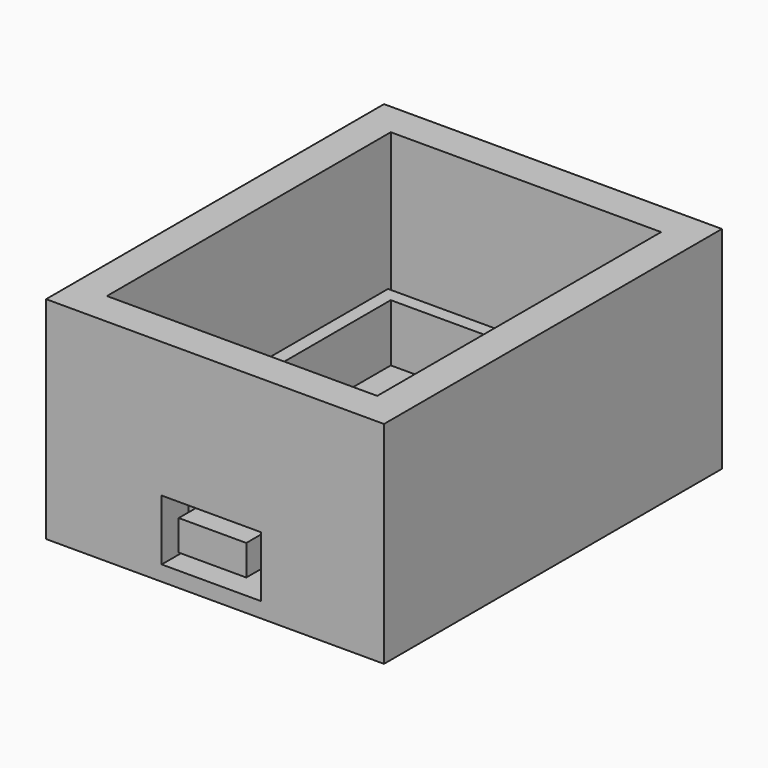
from build123d import *

# Parameters (mm, degrees)
F0_W      = 29.2
F0_H      = 37.7
F1_DEPTH  = 10
F2_T      = -1.6
F3_W      = 8
F3_H      = 3.6
F4_DEPTH  = 1.6
F5_W      = 4
F5_H      = 2.5
F6_DEPTH  = 1.6
F7_W      = 26
F7_H      = 34.5
F8_DEPTH  = 1.6
F9_W      = 32
F9_H      = 4
F9_W_2    = 4
F9_H_2    = 42
F10_DEPTH = 25
F11_W     = 40
F11_H     = 50
F11_W_2   = 32
F11_H_2   = 42
F12_DEPTH = 2
F13_W     = 11.7341736332
F13_H     = 7.1810703957
F13_W_2   = 8
F13_H_2   = 3.6
F14_DEPTH = 25


with BuildPart() as f1:
    # F0 (on Top) → F1 (new body)
    with BuildSketch(Plane.XY):
        Rectangle(F0_W, F0_H)
    extrude(amount=F1_DEPTH)

    # F2
    f2_openings = [f1.faces().sort_by_distance(p)[0] for p in [
        (0, 0, 10),
    ]]
    offset(amount=F2_T, openings=f2_openings)

    # F3 (on face) → F4 (cut, through all)
    with BuildSketch(Plane.XZ.offset(18.85)):
        with Locations((-0.3, 5.5)):
            Rectangle(F3_W, F3_H)
    extrude(amount=-F4_DEPTH, mode=Mode.SUBTRACT)

    # F5 (on face) → F6 (cut, through all)
    with BuildSketch(Plane(origin=(-14.6, 0, 0), x_dir=(0, -1, 0), z_dir=(-1, 0, 0))):
        with Locations((13.15, 4.95)):
            Rectangle(F5_W, F5_H)
    extrude(amount=-F6_DEPTH, mode=Mode.SUBTRACT)

    # F7 (on face) → F8 (join)
    with BuildSketch(Plane.XY.offset(1.6)):
        Rectangle(F7_W, F7_H)
    extrude(amount=F8_DEPTH)


with BuildPart() as f10:
    # F9 (on face) → F10 (new body)
    with BuildSketch(Plane(origin=(0, 0, 0), x_dir=(1, 0, 0), z_dir=(0, 0, -1))):
        with Locations((0, -23)):
            Rectangle(F9_W, F9_H)
        with Locations((-18, -23)):
            Rectangle(F9_W_2, F9_H)
        with Locations((18, -23)):
            Rectangle(F9_W_2, F9_H)
        with Locations((18, 23)):
            Rectangle(F9_W_2, F9_H)
        with Locations((18, 0)):
            Rectangle(F9_W_2, F9_H_2)
        with Locations((0, 23)):
            Rectangle(F9_W, F9_H)
        with Locations((-18, 23)):
            Rectangle(F9_W_2, F9_H)
        with Locations((-18, 0)):
            Rectangle(F9_W_2, F9_H_2)
    extrude(amount=-F10_DEPTH)

    # F11 (on face) → F12 (join)
    with BuildSketch(Plane(origin=(0, 0, 0), x_dir=(1, 0, 0), z_dir=(0, 0, -1))):
        Rectangle(F11_W, F11_H)
        Rectangle(F11_W_2, F11_H_2, mode=Mode.SUBTRACT)
        Rectangle(F11_W_2, F11_H_2)
    extrude(amount=-F12_DEPTH)

    # F13 (on face) → F14 (cut)
    with BuildSketch(Plane.XZ.offset(18.85)):
        with Locations((-0.450883992, 5.3956854972)):
            Rectangle(F13_W, F13_H)
        with Locations((-0.3, 5.5)):
            Rectangle(F13_W_2, F13_H_2, mode=Mode.SUBTRACT)
    extrude(amount=F14_DEPTH, mode=Mode.SUBTRACT)


solid = Compound([f1.part, f10.part])
